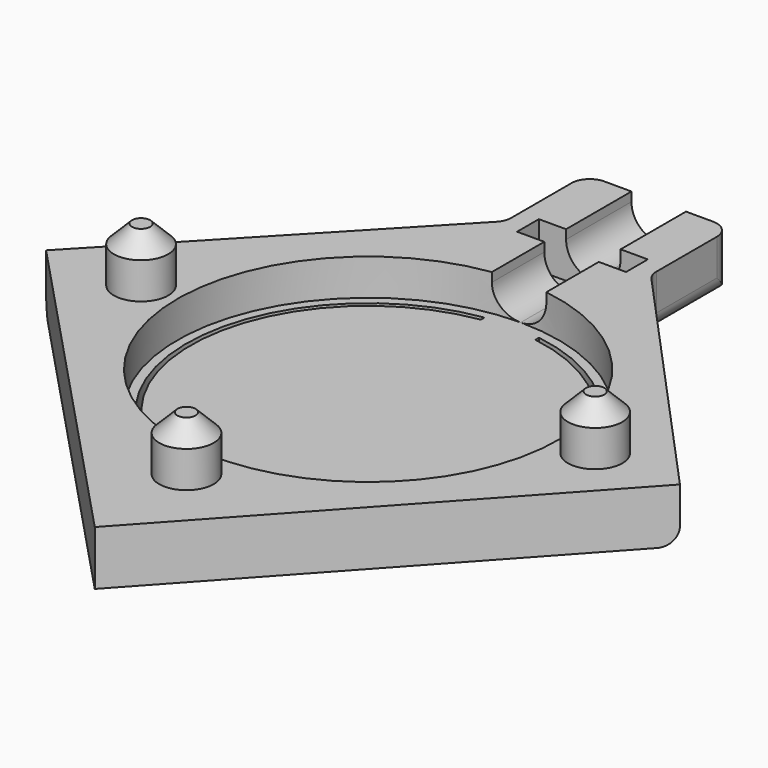
from build123d import *

# Parameters (mm, degrees)
F1_DEPTH  = 3
F3_DEPTH  = 2
F4_R      = 1.5
F5_DEPTH  = 3
F6_SIZE   = 1
F7_R      = 1
F9_DEPTH  = 1.0010001
F10_R     = 1.49999
F11_W     = 6
F11_H     = 1.5
F12_DEPTH = 2.5


# Not quite as in the source:
# - a fillet or chamfer is up to 0.001 mm smaller than in the source, because OpenCascade refuses the exact size


with BuildPart() as f1:
    # F0 (on Top) → F1 (new body)
    with BuildSketch(Plane.XY):
        Polygon((4, 20), (-4, 20), (-4, 14.4568322948), (-17.7288018167, 0), (0, -18.8113879412), (17.1686839312, 0), (4, 14.4568322948), align=None)
    extrude(amount=F1_DEPTH)

    # F2 (on face) → F3 (cut)
    with BuildSketch(Plane.XY.offset(3)):
        with BuildLine():
            Line((1.5, 20), (-1.5, 20))
            Line((-1.5, 20), (-1.5, 10.3923048454))
            ThreePointArc((-1.5, 10.3923048454), (0, -10.5), (1.5, 10.3923048454))
            Line((1.5, 10.3923048454), (1.5, 20))
        make_face()
    extrude(amount=-F3_DEPTH, mode=Mode.SUBTRACT)

    # F4 (on face) → F5 (join)
    with BuildSketch(Plane.XY.offset(3)):
        with Locations((12.5, 0)):
            Circle(F4_R)
        with Locations((-12.5, 0)):
            Circle(F4_R)
        with Locations((0, -12.5)):
            Circle(F4_R)
    extrude(amount=F5_DEPTH)

    # F6
    f6_edges = [f1.edges().sort_by_distance(p)[0] for p in [
        (-14, 0, 6),
        (-1.5, -12.5, 6),
        (11, 0, 6),
    ]]
    chamfer(f6_edges, length=F6_SIZE)

    # F7
    f7_edges = [f1.edges().sort_by_distance(p)[0] for p in [
        (4, 17.228416, 0),
        (-4, 17.228416, 0),
        (-4, 14.456832, 1.5),
        (-10.864401, 7.228416, 0),
        (-4, 20, 1.5),
        (4, 14.456832, 1.5),
        (10.584342, 7.228416, 0),
        (4, 20, 1.5),
    ]]
    fillet(f7_edges, radius=F7_R)

    # F8 (on face) → F9 (cut, through all)
    with BuildSketch(Plane.XY.offset(1)):
        with BuildLine():
            Line((-1.5, 9.633924434), (-1.5, 9.8868599666))
            ThreePointArc((-1.5, 9.8868599666), (0, -10), (1.5, 9.8868599666))
            Line((1.5, 9.8868599666), (1.5, 9.633924434))
            ThreePointArc((1.5, 9.633924434), (0, -9.75), (-1.5, 9.633924434))
        make_face()
    extrude(amount=-F9_DEPTH, mode=Mode.SUBTRACT)

    # F10 (radius 1.5 in the source; OpenCascade refuses exactly that, so slightly less here)
    f10_edges = [f1.edges().sort_by_distance(p)[0] for p in [
        (1.5, 15.196152, 1),
        (-1.5, 15.196152, 1),
    ]]
    fillet(f10_edges, radius=F10_R)

    # F11 (on face) → F12 (cut)
    with BuildSketch(Plane.XY.offset(3)):
        with Locations((0, 14.75)):
            Rectangle(F11_W, F11_H)
    extrude(amount=-F12_DEPTH, mode=Mode.SUBTRACT)


solid = f1.part
